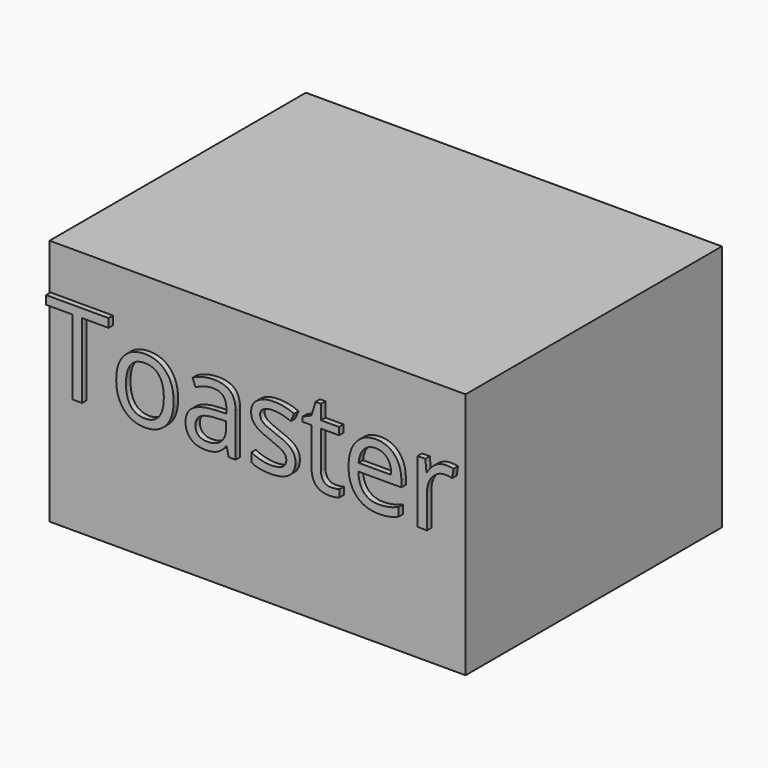
from build123d import *

# Parameters (mm, degrees)
F0_W         = 469.9
F0_H         = 279.4
F1_DEPTH     = 361.95
F2_TEXT_SIZE = 131.86705253
F3_DEPTH     = 6.35


# Not quite as in the source:
# - Text() gives the source's letters only with a copy of the font that has no kerning and outlines rounded to 1/6400 em; it was checked with that copy


with BuildPart() as f1:
    # F0 (on Front) → F1 (new body)
    with BuildSketch(Plane.XZ):
        with Locations((234.95, 139.7)):
            Rectangle(F0_W, F0_H)
    extrude(amount=F1_DEPTH)


with BuildPart() as f3:
    # F2 (on face) → F3 (new body)
    with BuildSketch(Plane.XZ.offset(361.95)):
        with Locations((0, 134.1574607893)):
            Text('Toaster', F2_TEXT_SIZE, font='Open Sans', text_align=(TextAlign.LEFT, TextAlign.BOTTOM))
    extrude(amount=F3_DEPTH)


solid = Compound([f1.part, f3.part])
